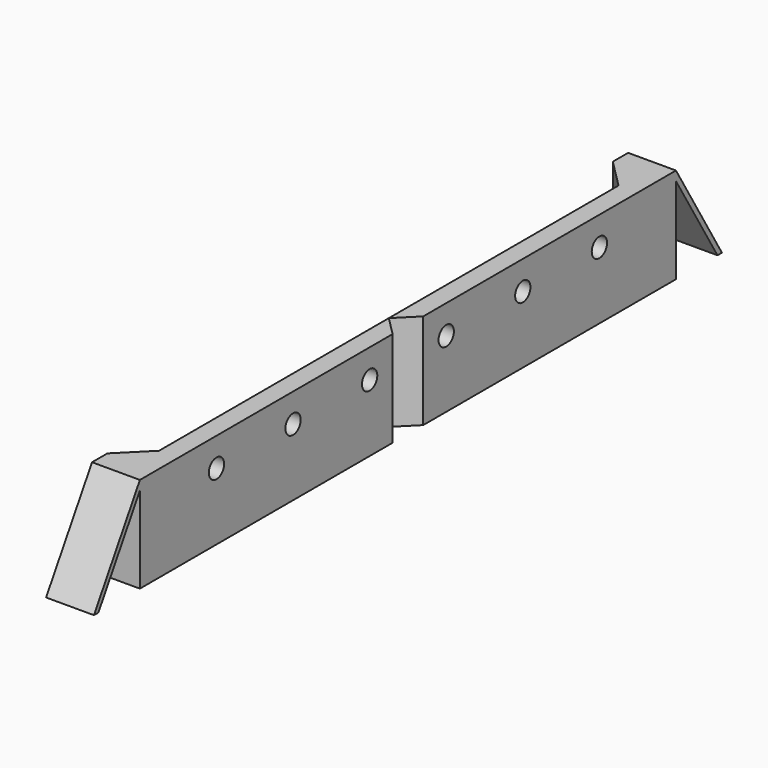
from build123d import *

# Parameters (mm, degrees)
F1_DEPTH  = 10
F2_W      = 2
F2_H      = 10
F3_DEPTH  = 25
F4_DEPTH  = 44.001
F6_DEPTH  = 41.001
F9_DEPTH  = 3
F10_SIZE  = 2.99999
F12_DEPTH = 3
F13_SIZE  = 2.99999
F16_D     = 2
F17_D     = 2
F18_DEPTH = 25
F21_DEPTH = 25


# Not quite as in the source:
# - a fillet or chamfer is up to 0.001 mm smaller than in the source, because OpenCascade refuses the exact size
# - a feature of the source that left no trace in its solid (it failed there, or was rolled back) is left out


with BuildPart() as f1:
    # F0 (on Top) → F1 (new body)
    with BuildSketch(Plane.XY):
        Polygon((-22, -19.5), (-20, -19.5), (-20, 19.5), (20, 19.5), (20, 21.5), (-22, 21.5), align=None)
        Polygon((20, 19.5), (20, -19.5), (-20, -19.5), (-22, -19.5), (-22, -21.5), (22, -21.5), (22, 21.5), (20, 21.5), align=None)
    extrude(amount=-F1_DEPTH)

    # F2 (on face) → F3 (cut)
    with BuildSketch(Plane(origin=(-22, 0, 0), x_dir=(0, -1, 0), z_dir=(-1, 0, 0))):
        Polygon((19.5, 0), (13.5, 0), (19.5, -10), align=None)
        with Locations((20.5, -5)):
            Rectangle(F2_W, F2_H)
        Polygon((13.5, -10), (18.9169048105, -10), (13.5, -0.9718253158), align=None)
    extrude(amount=-F3_DEPTH, mode=Mode.SUBTRACT)

    # F2 (on face) → F4 (cut, through all)
    with BuildSketch(Plane(origin=(-22, 0, 0), x_dir=(0, -1, 0), z_dir=(-1, 0, 0))):
        Polygon((19.5, 0), (13.5, 0), (19.5, -10), align=None)
        with Locations((20.5, -5)):
            Rectangle(F2_W, F2_H)
    extrude(amount=-F4_DEPTH, mode=Mode.SUBTRACT)

    # F5 (on face) → F6 (cut, through all)
    with BuildSketch(Plane(origin=(0, 21.5, 0), x_dir=(-1, 0, 0), z_dir=(0, 1, 0))):
        Polygon((-14, -0.9077913453), (-20, -10), (-14, -10), align=None)
        Polygon((-22, -10), (-20, -10), (-20, -9.0922086547), (-14, 0), (-22, 0), align=None)
    extrude(amount=-F6_DEPTH, mode=Mode.SUBTRACT)

    # F8 (on face) → F9 (join)
    with BuildSketch(Plane(origin=(0, 21.5, 0), x_dir=(-1, 0, 0), z_dir=(0, 1, 0))):
        Polygon((-14, -10), (-9, -10), (-9, 0), (-14, 0), (-20, -9.0922086547), (-20, -10), (-14, -0.9077913453), align=None)
    extrude(amount=F9_DEPTH)

    # F10 (size 3 in the source; OpenCascade refuses exactly that, so slightly less here)
    f10_edges = [f1.edges().sort_by_distance(p)[0] for p in [
        (9, 24.5, -5),
    ]]
    chamfer(f10_edges, length=F10_SIZE)

    # F11 (on face) → F12 (join)
    with BuildSketch(Plane(origin=(-22, 0, 0), x_dir=(0, -1, 0), z_dir=(-1, 0, 0))):
        Polygon((13.5, 0), (8.5, 0), (8.5, -10), (13.5, -10), (13.5, -0.9718253158), (18.9169048105, -10), (19.5, -10), align=None)
    extrude(amount=F12_DEPTH)

    # F13 (size 3 in the source; OpenCascade refuses exactly that, so slightly less here)
    f13_edges = [f1.edges().sort_by_distance(p)[0] for p in [
        (-25, -8.5, -5),
    ]]
    chamfer(f13_edges, length=F13_SIZE)

    # F16 (through all)
    with Locations(Plane(origin=(-22, 0, 0), x_dir=(0, -1, 0), z_dir=(-1, 0, 0))):
        with Locations((-6.5, -3), (3.5, -3), (-16.5, -3)):
            Hole(F16_D / 2)

    # F17 (through all)
    with Locations(Plane(origin=(0, 21.5, 0), x_dir=(-1, 0, 0), z_dir=(0, 1, 0))):
        with Locations((-3.5, -3), (6.5, -3), (16.5, -3)):
            Hole(F17_D / 2)

    # F18 (cut): a face of the model
    f18_faces = [f1.faces().sort_by_distance(p)[0] for p in [
        (-2.5776416517, 19.5, -5.0560962008),
    ]]
    extrude(f18_faces, amount=-F18_DEPTH, mode=Mode.SUBTRACT)

    # F19: F1 across face


with BuildPart() as f1_1:
    add(f1.part)
    add(f1.part.mirror(Plane(origin=(-21, 21.5, -5), x_dir=(-1, 0, 0), z_dir=(0, 1, 0))))

    # F20 (on face) → F21 (cut)
    with BuildSketch(Plane.XY):
        Polygon((-20, 23.5), (-22, 21.5), (-20, 19.5), align=None)
    extrude(amount=-F21_DEPTH, mode=Mode.SUBTRACT)


solid = f1_1.part
